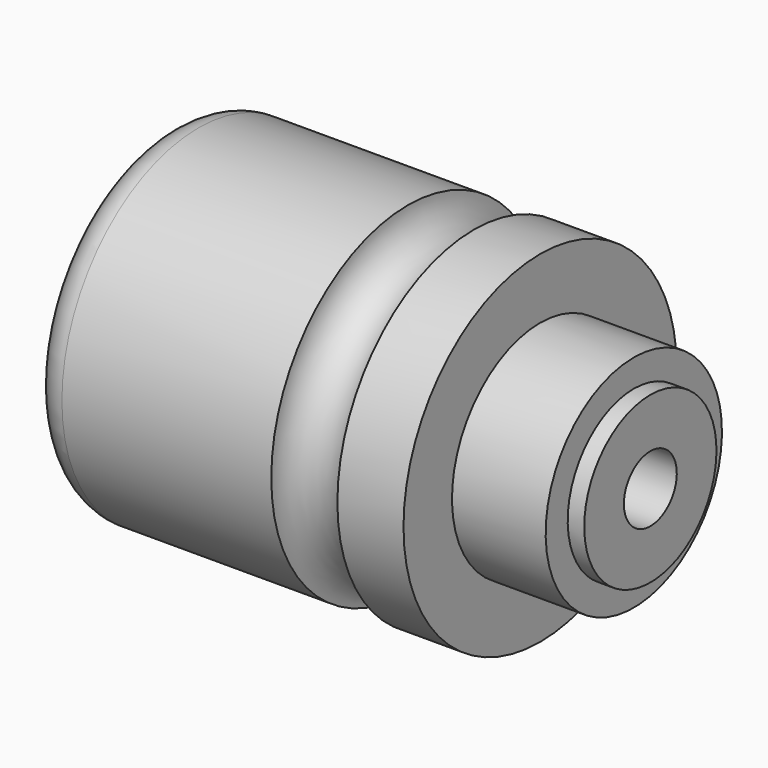
from build123d import *

# Parameters (mm, degrees)
F4_R = 5.99999


# Not quite as in the source:
# - a fillet or chamfer is up to 0.001 mm smaller than in the source, because OpenCascade refuses the exact size


with BuildPart() as f1:
    # F0 (on Front) → F1 (revolve)
    with BuildSketch(Plane.XZ):
        with BuildLine():
            Line((0, 31), (0, 0))
            Line((0, 0), (88, 0))
            Line((88, 0), (88, 15))
            Line((88, 15), (85, 15))
            Line((85, 15), (85, 20))
            Line((85, 20), (68, 20))
            Line((68, 20), (68, 31))
            Line((68, 31), (56, 31))
            ThreePointArc((56, 31), (50, 25), (44, 31))
            Line((44, 31), (0, 31))
        make_face()
    revolve(axis=Axis((57.4120017065, 0, 0), (1, 0, 0)))

    # F2 (on Front) → F3 (revolve, cut)
    with BuildSketch(Plane.XZ):
        Polygon((0, 25), (0, 0), (88, 0), (88, 6), (30, 6), (30, 16), (22, 16), (22, 20.5), (15, 20.5), (15, 12.5), (12, 12.5), (12, 16), (1.5, 16), (1.5, 25), align=None)
    revolve(axis=Axis((-12.9248626642, 0, 0), (-1, 0, 0)), mode=Mode.SUBTRACT)

    # F4 (radius 6 in the source; OpenCascade refuses exactly that, so slightly less here)
    f4_edges = [f1.edges().sort_by_distance(p)[0] for p in [
        (0, 0, -31),
    ]]
    fillet(f4_edges, radius=F4_R)


solid = f1.part
